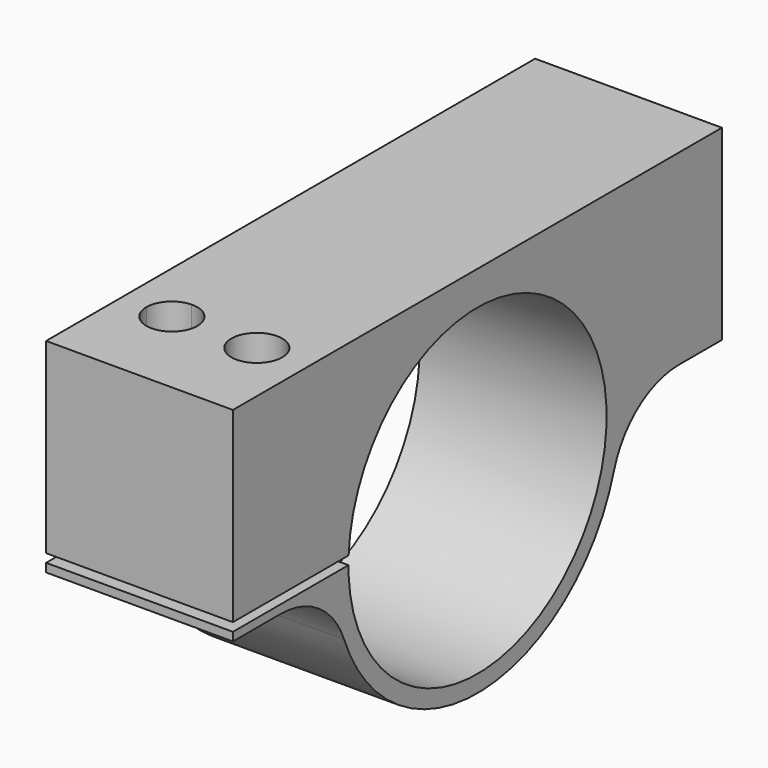
from build123d import *

# Parameters (mm, degrees)
F1_DEPTH     = 22
F3_DEPTH     = 25
F4_DEPTH     = 11
F5_R         = 1.75
F6_DEPTH     = 20
F7_T1_DEPTH  = 22
F7_T6_DEPTH  = 22
F7_S7_R      = 1.75
F7_T8_DEPTH  = 14
F7_S9_R      = 1.75
F7_T10_DEPTH = 14


# Not quite as in the source:
# - a fillet or chamfer that OpenCascade refuses, or shapes differently, is made with other operations: its cross-section is extruded or revolved along the edge and cut away or added
# - after a boolean that leaves OpenCascade's solid faulty, fix() repairs it


with BuildPart() as f1:
    # F0 (on Right) → F1 (new body)
    with BuildSketch(Plane.YZ):
        with BuildLine():
            ThreePointArc((-20.9761769634, 1), (0, 21), (20.9761769634, 1))
            Line((20.9761769634, 1), (35.9761769634, 1))
            Line((35.9761769634, 1), (35.9761769634, 23))
            Line((35.9761769634, 23), (-36, 23))
            Line((-36, 23), (-36, 1))
            Line((-36, 1), (-20.9761769634, 1))
        make_face()
        with BuildLine():
            ThreePointArc((-18.973665961, -1), (-18.9934153493, -0.5001733404), (-19, 0))
            Line((-19, 0), (-21, 0))
            ThreePointArc((-21, 0), (-20.9940433961, -0.5001418641), (-20.9761769634, -1))
            Line((-20.9761769634, -1), (-18.973665961, -1))
        make_face()
        with BuildLine():
            ThreePointArc((18.973665961, 1), (1, -18.973665961), (-18.973665961, -1))
            Line((-18.973665961, -1), (-20.9761769634, -1))
            ThreePointArc((-20.9761769634, -1), (1, -20.9761769634), (20.9761769634, 1))
            Line((20.9761769634, 1), (18.973665961, 1))
        make_face()
        with BuildLine():
            ThreePointArc((-18.973665961, 1), (0, 19), (18.973665961, 1))
            Line((18.973665961, 1), (20.9761769634, 1))
            ThreePointArc((20.9761769634, 1), (0, 21), (-20.9761769634, 1))
            Line((-20.9761769634, 1), (-18.973665961, 1))
        make_face()
        with BuildLine():
            ThreePointArc((-20.9761769634, -1), (-20.9940433961, -0.5001418641), (-21, 0))
            Line((-21, 0), (-36, 0))
            Line((-36, 0), (-36, -1))
            Line((-36, -1), (-20.9761769634, -1))
        make_face()
    extrude(amount=F1_DEPTH)

    # F2 (on face) → F3 (cut)
    with BuildSketch(Plane.XY.offset(23)):
        with BuildLine():
            ThreePointArc((4.25, -24.9799919936), (6, -26.7299919936), (7.75, -24.9799919936))
            Line((7.75, -24.9799919936), (6, -24.9799919936))
            Line((6, -24.9799919936), (4.25, -24.9799919936))
        make_face()
        with BuildLine():
            Line((6, -24.9799919936), (5.93, -23.231392554))
            ThreePointArc((5.93, -23.231392554), (4.7380570536, -23.7675564283), (4.25, -24.9799919936))
            Line((4.25, -24.9799919936), (6, -24.9799919936))
        make_face()
        with BuildLine():
            Line((6, -24.9799919936), (7.75, -24.9799919936))
            ThreePointArc((7.75, -24.9799919936), (7.2124355653, -23.7180490472), (5.93, -23.231392554))
            Line((5.93, -23.231392554), (6, -24.9799919936))
        make_face()
        with BuildLine():
            ThreePointArc((17.75, -24.9799919936), (16, -23.2299919936), (14.25, -24.9799919936))
            ThreePointArc((14.25, -24.9799919936), (16, -26.7299919936), (17.75, -24.9799919936))
        make_face()
    extrude(amount=-F3_DEPTH, mode=Mode.SUBTRACT)

    # F2 (on face) → F4 (cut)
    with BuildSketch(Plane.XY.offset(23)):
        with BuildLine():
            Line((9, -24.9799919936), (7.75, -24.9799919936))
            ThreePointArc((7.75, -24.9799919936), (6, -26.7299919936), (4.25, -24.9799919936))
            Line((4.25, -24.9799919936), (3, -24.9799919936))
            ThreePointArc((3, -24.9799919936), (6, -27.9799919936), (9, -24.9799919936))
        make_face()
        with BuildLine():
            ThreePointArc((4.25, -24.9799919936), (4.7380570536, -23.7675564283), (5.93, -23.231392554))
            Line((5.93, -23.231392554), (5.88, -21.9823929544))
            ThreePointArc((5.88, -21.9823929544), (3.8366692347, -22.9015310245), (3, -24.9799919936))
            Line((3, -24.9799919936), (4.25, -24.9799919936))
        make_face()
        with BuildLine():
            ThreePointArc((5.93, -23.231392554), (7.2124355653, -23.7180490472), (7.75, -24.9799919936))
            Line((7.75, -24.9799919936), (9, -24.9799919936))
            ThreePointArc((9, -24.9799919936), (8.0784609691, -22.8166612283), (5.88, -21.9823929544))
            Line((5.88, -21.9823929544), (5.93, -23.231392554))
        make_face()
        with BuildLine():
            ThreePointArc((19, -24.9799919936), (16, -21.9799919936), (13, -24.9799919936))
            ThreePointArc((13, -24.9799919936), (16, -27.9799919936), (19, -24.9799919936))
        make_face()
        with BuildLine():
            ThreePointArc((17.75, -24.9799919936), (16, -26.7299919936), (14.25, -24.9799919936))
            ThreePointArc((14.25, -24.9799919936), (16, -23.2299919936), (17.75, -24.9799919936))
        make_face(mode=Mode.SUBTRACT)
    extrude(amount=-F4_DEPTH, mode=Mode.SUBTRACT)

    # F7: fillet of radius 10 on 2 edges, made by hand

    # F7_s2 → F7_t1 (join)
    with BuildSketch(Plane.YZ):
        with BuildLine():
            ThreePointArc((29.6647939484, 1), (23.7079599766, -0.967806711), (20.095505578, -6.0967741935))
            ThreePointArc((20.095505578, -6.0967741935), (20.8401494161, -2.5861500957), (20.9761769634, 1))
            Line((20.9761769634, 1), (29.6647939484, 1))
        make_face()
    extrude(amount=F7_T1_DEPTH)


with BuildPart() as f6:
    # F5 (on face) → F6 (new body)
    with BuildSketch(Plane(origin=(0, 0, -1), x_dir=(1, 0, 0), z_dir=(0, 0, -1))):
        Polygon((19.897114317, 27.2299919936), (16, 29.4799919936), (12.102885683, 27.2299919936), (12.102885683, 22.7299919936), (15.1405824223, 20.9761769634), (16.8594175777, 20.9761769634), (19.897114317, 22.7299919936), align=None)
        with Locations((16, 24.9799919936)):
            Circle(F5_R, mode=Mode.SUBTRACT)
    extrude(amount=F6_DEPTH)


with BuildPart() as f6b:
    # F5 (on face) → F6, piece 2 (new body)
    with BuildSketch(Plane(origin=(0, 0, -1), x_dir=(1, 0, 0), z_dir=(0, 0, -1))):
        Polygon((5.1405824223, 20.9761769634), (6.8594175777, 20.9761769634), (9.897114317, 22.7299919936), (9.897114317, 27.2299919936), (6, 29.4799919936), (2.102885683, 27.2299919936), (2.102885683, 22.7299919936), align=None)
        with Locations((6, 24.9799919936)):
            Circle(F5_R, mode=Mode.SUBTRACT)
    extrude(amount=F6_DEPTH)


with BuildPart() as f7_tool4:
    # F7_s5 → F7_t6 (new body)
    with BuildSketch(Plane.YZ):
        with BuildLine():
            ThreePointArc((-28.9827534924, -1), (-23.3031351499, -2.7694510825), (-19.6334781723, -7.4516129032))
            ThreePointArc((-19.6334781723, -7.4516129032), (-20.5594710492, -4.2788024233), (-20.9761769634, -1))
            Line((-20.9761769634, -1), (-28.9827534924, -1))
        make_face()
    extrude(amount=F7_T6_DEPTH)

    # F7_s7 → F7_t8 (cut, symmetric)
    with BuildSketch(Plane.XY.offset(-4.2)):
        with Locations((16, -24.9799919936)):
            Circle(F7_S7_R)
    extrude(amount=F7_T8_DEPTH, both=True, mode=Mode.SUBTRACT)

    # F7_s9 → F7_t10 (cut, symmetric)
    with BuildSketch(Plane.XY.offset(-4.2)):
        with Locations((6, -24.9799919936)):
            Circle(F7_S9_R)
    extrude(amount=F7_T10_DEPTH, both=True, mode=Mode.SUBTRACT)


with BuildPart() as f1_1:
    add(f1.part)

    # F7_t3: union F7_tool4
    add(f7_tool4.part)

    # F8: cut F6, F6b
    add(f6.part, mode=Mode.SUBTRACT)
    add(f6b.part, mode=Mode.SUBTRACT)

    add(f1_1.part.fix(), mode=Mode.REPLACE)


solid = f1_1.part
